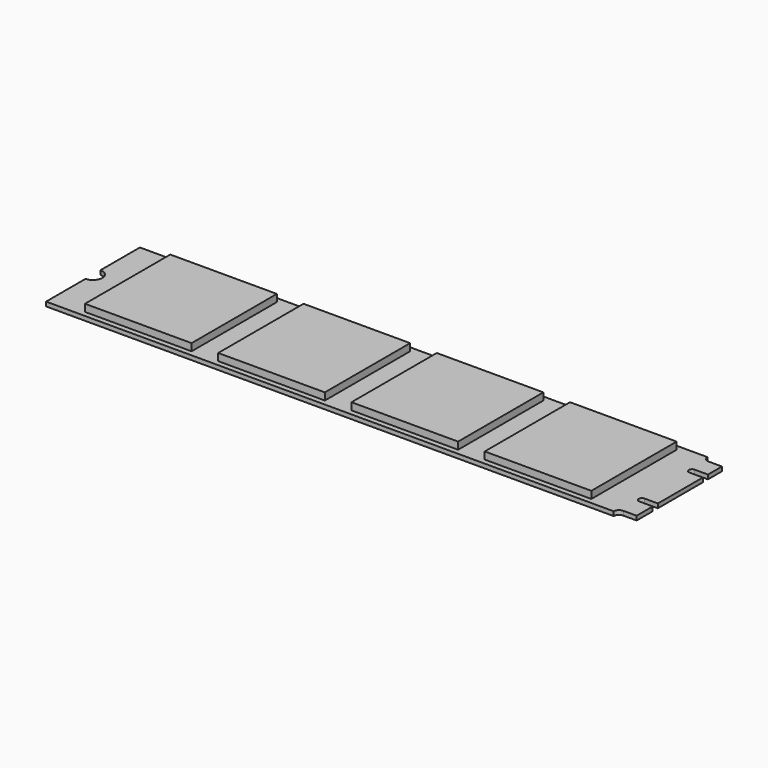
from build123d import *

# Parameters (mm, degrees)
F0_W     = 110
F0_H     = 22
F1_DEPTH = 0.8
F2_W     = 3.5
F2_H     = 1
F2_W_2   = 2.5
F2_H_2   = 1.2
F3_DEPTH = 0.801
F4_R     = 0.99999
F2_W_3   = 20
F2_H_3   = 20
F5_DEPTH = 1.35


# Not quite as in the source:
# - a fillet or chamfer is up to 0.001 mm smaller than in the source, because OpenCascade refuses the exact size


with BuildPart() as f1:
    # F0 (on Top) → F1 (new body)
    with BuildSketch(Plane.XY):
        Rectangle(F0_W, F0_H)
    extrude(amount=F1_DEPTH)

    # F2 (on face) → F3 (cut, through all)
    with BuildSketch(Plane.XY.offset(0.8)):
        with BuildLine():
            Line((-55, 1.75), (-55, -1.75))
            ThreePointArc((-55, -1.75), (-53.25, 0), (-55, 1.75))
        make_face()
        with Locations((53.25, 10.5)):
            Rectangle(F2_W, F2_H)
        with Locations((53.25, -10.5)):
            Rectangle(F2_W, F2_H)
        with BuildLine():
            ThreePointArc((52.5, -5.025), (51.9, -5.625), (52.5, -6.225))
            Line((52.5, -6.225), (52.5, -5.025))
        make_face()
        with BuildLine():
            Line((52.5, 5.525), (52.5, 6.725))
            ThreePointArc((52.5, 6.725), (51.9, 6.125), (52.5, 5.525))
        make_face()
        with Locations((53.75, -5.625)):
            Rectangle(F2_W_2, F2_H_2)
        with Locations((53.75, 6.125)):
            Rectangle(F2_W_2, F2_H_2)
    extrude(amount=-F3_DEPTH, mode=Mode.SUBTRACT)

    # F4 (radius 1 in the source; OpenCascade refuses exactly that, so slightly less here)
    f4_edges = [f1.edges().sort_by_distance(p)[0] for p in [
        (51.5, -10, 0.4),
        (51.5, 10, 0.4),
    ]]
    fillet(f4_edges, radius=F4_R)

    # F2 (on face) → F5 (join)
    with BuildSketch(Plane.XY.offset(0.8)):
        with Locations((36.5, 0)):
            Rectangle(F2_W_3, F2_H_3)
        with Locations((11.5, 0)):
            Rectangle(F2_W_3, F2_H_3)
        with Locations((-13.5, 0)):
            Rectangle(F2_W_3, F2_H_3)
        with Locations((-38.5, 0)):
            Rectangle(F2_W_3, F2_H_3)
    extrude(amount=F5_DEPTH)


solid = f1.part
